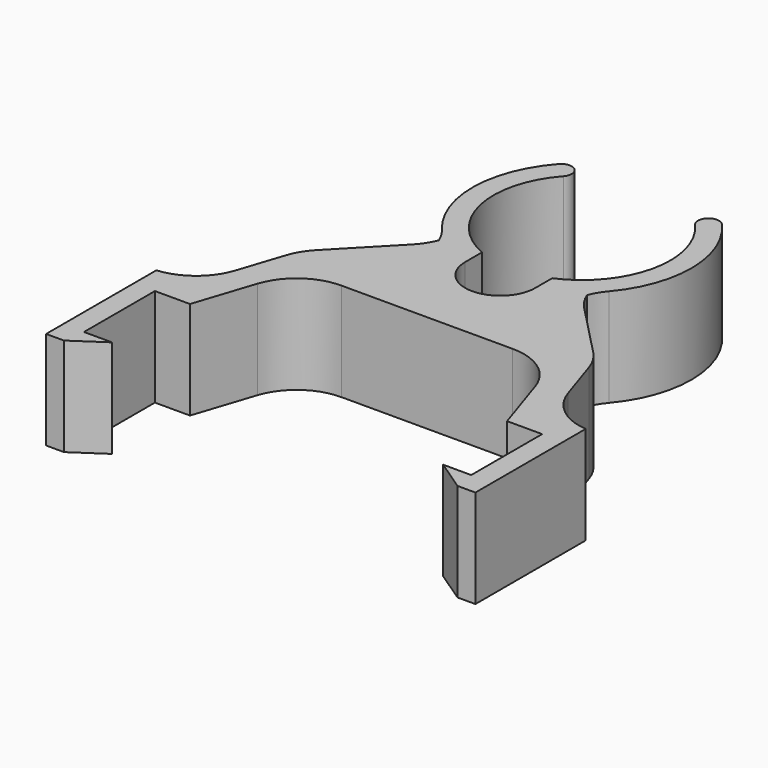
from build123d import *

# Parameters (mm, degrees)
F1_DEPTH    = 4.445
F5_DEPTH    = 4.445
F6_W        = 6.35
F6_H        = 1.905
F7_DEPTH    = 8.891
F8_T1_DEPTH = 8.89
F8_T3_DEPTH = 14.7171591693


# Not quite as in the source:
# - a fillet or chamfer that OpenCascade refuses, or shapes differently, is made with other operations: its cross-section is extruded or revolved along the edge and cut away or added
# - a feature names something its author has since deleted; it is built from what else it names


with BuildPart() as f1:
    # F0 (on Top) → F1 (new body, symmetric)
    with BuildSketch(Plane.XY):
        with BuildLine():
            ThreePointArc((5.9581914894, 5.3400332561), (0, -8.001), (-5.9581914894, 5.3400332561))
            ThreePointArc((-5.9581914894, 5.3400332561), (-6.0317817552, 6.6850600115), (-7.3768085106, 6.6114697456))
            ThreePointArc((-7.3768085106, 6.6114697456), (-9.880255326, -0.7137161157), (-6.35, -7.6030478099))
            Line((-6.35, -7.6030478099), (-6.35, -15.621))
            Line((-6.35, -15.621), (6.35, -15.621))
            Line((6.35, -15.621), (6.35, -7.6030478099))
            ThreePointArc((6.35, -7.6030478099), (9.880255326, -0.7137161157), (7.3768085106, 6.6114697456))
            ThreePointArc((7.3768085106, 6.6114697456), (6.0317817552, 6.6850600115), (5.9581914894, 5.3400332561))
        make_face()
    extrude(amount=F1_DEPTH, both=True)

    # F4 (on Top) → F5 (join, symmetric)
    with BuildSketch(Plane.XY):
        Polygon((-16.1900234303, -23.876), (-19.431, -23.876), (-19.431, -36.3474), (-17.810278645, -36.3474), (-14.986, -34.4424), (-17.526, -34.4424), (-17.526, -26.416), (-14.351, -26.416), (-11.43, -17.526), (0, -17.526), (11.43, -17.526), (14.351, -26.416), (17.526, -26.416), (17.526, -34.4424), (14.986, -34.4424), (17.810278645, -36.3474), (19.431, -36.3474), (19.431, -23.876), (16.1900234303, -23.876), (13.354690472, -15.2467257791), (6.35, -8.001), (-6.35, -8.001), (-13.354690472, -15.2467257791), align=None)
    extrude(amount=F5_DEPTH, both=True)

    # F6 (on face) → F7 (cut, through all)
    with BuildSketch(Plane.XY.offset(4.445)):
        with Locations((0, -8.2965708058)):
            Rectangle(F6_W, F6_H)
        with BuildLine():
            Line((3.175, -9.2490708058), (-3.175, -9.2490708058))
            ThreePointArc((-3.175, -9.2490708058), (0, -12.4240708058), (3.175, -9.2490708058))
        make_face()
    extrude(amount=-F7_DEPTH, mode=Mode.SUBTRACT)

    # F8: fillet of radius 5.08 on 10 edges, made by hand

    # F8_s2 → F8_t1 (join)
    with BuildSketch(Plane.XY.offset(-4.445)):
        with BuildLine():
            ThreePointArc((15.0482804654, -20.4011301068), (16.7183588568, -22.7960371716), (19.431, -23.876))
            Line((19.431, -23.876), (16.1900234303, -23.876))
            Line((16.1900234303, -23.876), (15.0482804654, -20.4011301068))
        make_face()
        with BuildLine():
            ThreePointArc((-19.431, -23.876), (-16.7183588568, -22.7960371716), (-15.0482804654, -20.4011301068))
            Line((-15.0482804654, -20.4011301068), (-16.1900234303, -23.876))
            Line((-16.1900234303, -23.876), (-19.431, -23.876))
        make_face()
        with BuildLine():
            ThreePointArc((-7.7776621969, -9.4777888496), (-6.7204206111, -7.8512238682), (-6.35, -5.9469492084))
            Line((-6.35, -5.9469492084), (-6.35, -8.001))
            Line((-6.35, -8.001), (-7.7776621969, -9.4777888496))
        make_face()
        with BuildLine():
            ThreePointArc((6.35, -5.9469492084), (6.7204206111, -7.8512238682), (7.7776621969, -9.4777888496))
            Line((7.7776621969, -9.4777888496), (6.35, -8.001))
            Line((6.35, -8.001), (6.35, -5.9469492084))
        make_face()
        with BuildLine():
            ThreePointArc((7.5554237288, -6.4065910029), (6.6608676126, -7.9422290783), (6.35, -9.6920222864))
            Line((6.35, -9.6920222864), (6.35, -7.6030478099))
            ThreePointArc((6.35, -7.6030478099), (6.9784009266, -7.0307009969), (7.5554237288, -6.4065910029))
        make_face()
        with BuildLine():
            ThreePointArc((-6.35, -9.6920222864), (-6.6608676126, -7.9422290783), (-7.5554237288, -6.4065910029))
            ThreePointArc((-7.5554237288, -6.4065910029), (-6.9784009266, -7.0307009969), (-6.35, -7.6030478099))
            Line((-6.35, -7.6030478099), (-6.35, -9.6920222864))
        make_face()
        with BuildLine():
            ThreePointArc((-7.7519531394, -17.526), (-10.7311180697, -18.4912732389), (-12.5781144245, -21.020261292))
            Line((-12.5781144245, -21.020261292), (-11.43, -17.526))
            Line((-11.43, -17.526), (-7.7519531394, -17.526))
        make_face()
        with BuildLine():
            ThreePointArc((12.5781144245, -21.020261292), (10.7311180697, -18.4912732389), (7.7519531394, -17.526))
            Line((7.7519531394, -17.526), (11.43, -17.526))
            Line((11.43, -17.526), (12.5781144245, -21.020261292))
        make_face()
    extrude(amount=F8_T1_DEPTH)

    # F8_s4 → F8_t3 (cut)
    with BuildSketch(Plane.XY.offset(-7.3585795846)):
        with BuildLine():
            ThreePointArc((-13.718483852, -16.3539230226), (-13.2417008107, -15.3149124297), (-12.54466037, -14.4088220894))
            Line((-12.54466037, -14.4088220894), (-13.354690472, -15.2467257791))
            Line((-13.354690472, -15.2467257791), (-13.718483852, -16.3539230226))
        make_face()
        with BuildLine():
            ThreePointArc((12.54466037, -14.4088220894), (13.2417008107, -15.3149124297), (13.718483852, -16.3539230226))
            Line((13.718483852, -16.3539230226), (13.354690472, -15.2467257791))
            Line((13.354690472, -15.2467257791), (12.54466037, -14.4088220894))
        make_face()
    extrude(amount=F8_T3_DEPTH, mode=Mode.SUBTRACT)


solid = f1.part
